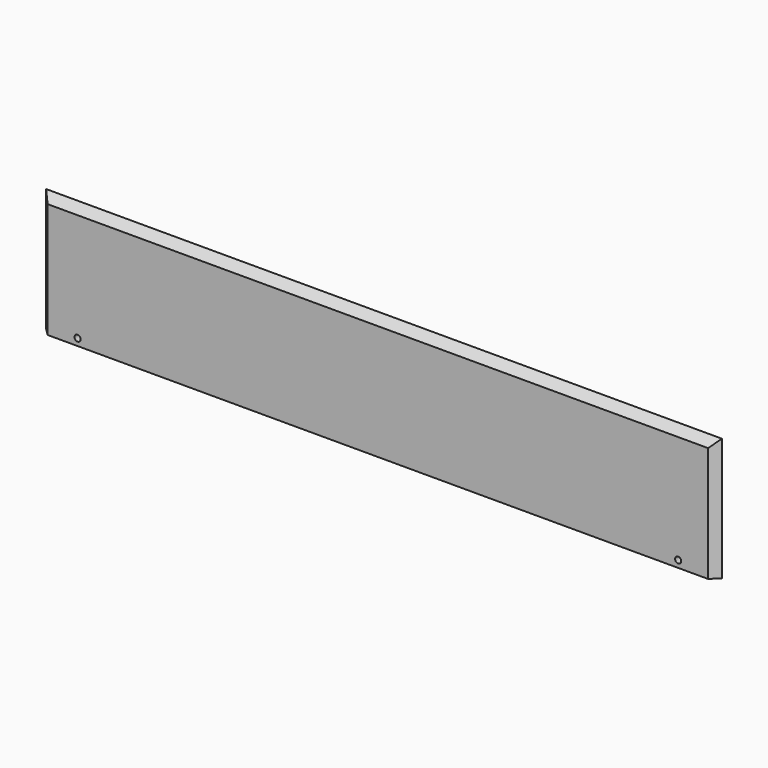
from build123d import *

# Parameters (mm, degrees)
F0_W     = 2200
F0_H     = 400
F1_DEPTH = 25
F2_R     = 10
F3_DEPTH = 25
F4_R     = 10
F5_DEPTH = 25
F6_DEPTH = 100
F7_DEPTH = 100
F8_SIZE  = 24.99999


# Not quite as in the source:
# - a fillet or chamfer is up to 0.001 mm smaller than in the source, because OpenCascade refuses the exact size


with BuildPart() as f1:
    # F0 (on Front) → F1 (new body)
    with BuildSketch(Plane.XZ):
        Rectangle(F0_W, F0_H)
    extrude(amount=F1_DEPTH)

    # F2 (on face) → F3 (cut)
    with BuildSketch(Plane.XZ.offset(25)):
        with Locations((977.5, -77.5)):
            Circle(F2_R)
    extrude(amount=-F3_DEPTH, mode=Mode.SUBTRACT)

    # F4 (on face) → F5 (cut)
    with BuildSketch(Plane.XZ.offset(25)):
        with Locations((-977.5, -77.5)):
            Circle(F4_R)
    extrude(amount=-F5_DEPTH, mode=Mode.SUBTRACT)

    # F6 (add): a face of the model
    f6_faces = [f1.faces().sort_by_distance(p)[0] for p in [
        (0, -12.5, 200),
    ]]
    extrude(f6_faces, amount=F6_DEPTH)

    # F7 (cut): a face of the model
    f7_faces = [f1.faces().sort_by_distance(p)[0] for p in [
        (0, -12.5, -200),
    ]]
    extrude(f7_faces, amount=-F7_DEPTH, mode=Mode.SUBTRACT)

    # F8 (size 25 in the source; OpenCascade refuses exactly that, so slightly less here)
    f8_edges = [f1.edges().sort_by_distance(p)[0] for p in [
        (-1100, -25, 100),
        (0, -25, 300),
        (1100, -25, 100),
    ]]
    chamfer(f8_edges, length=F8_SIZE)


solid = f1.part
